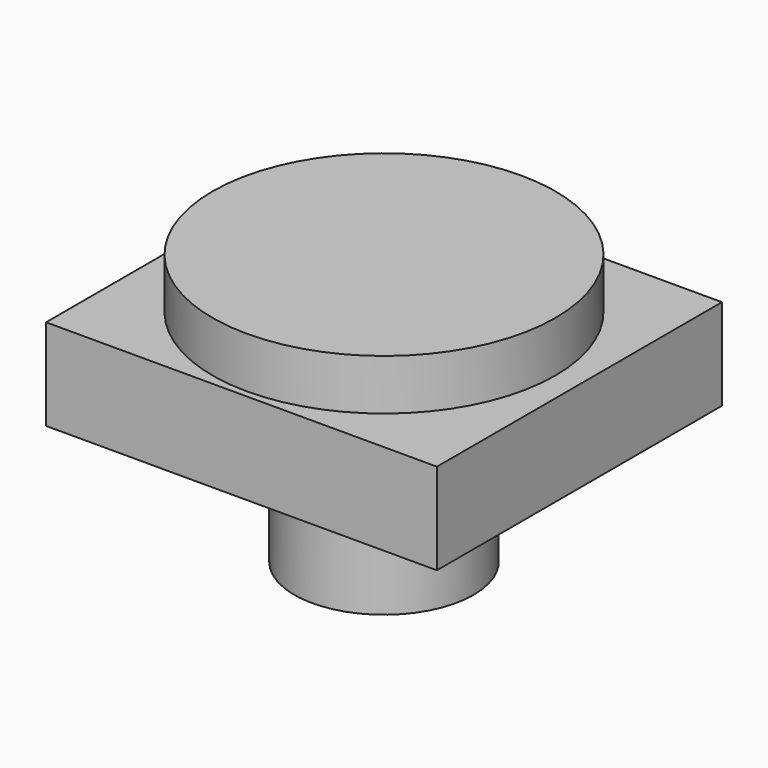
from build123d import *

# Parameters (mm, degrees)
F0_W     = 107.0966944098
F0_H     = 97.6227968931
F1_DEPTH = 25
F2_R     = 24.5699498699
F3_DEPTH = 25.001
F4_R     = 24.5699498699
F5_DEPTH = 60.2
F6_R     = 46.9734129042
F7_DEPTH = 13.9


with BuildPart() as f1:
    # F0 (on Top) → F1 (new body)
    with BuildSketch(Plane.XY):
        Rectangle(F0_W, F0_H)
    extrude(amount=F1_DEPTH)

    # F2 (on face) → F3 (cut, through all)
    with BuildSketch(Plane.XY.offset(25)):
        Circle(F2_R)
    extrude(amount=-F3_DEPTH, mode=Mode.SUBTRACT)


with BuildPart() as f5:
    # F4 (on face) → F5 (new body)
    with BuildSketch(Plane.XY.offset(25)):
        Circle(F4_R)
    extrude(amount=-F5_DEPTH)

    # F6 (on face) → F7 (join)
    with BuildSketch(Plane.XY.offset(25)):
        Circle(F6_R)
    extrude(amount=F7_DEPTH)


solid = Compound([f1.part, f5.part])
